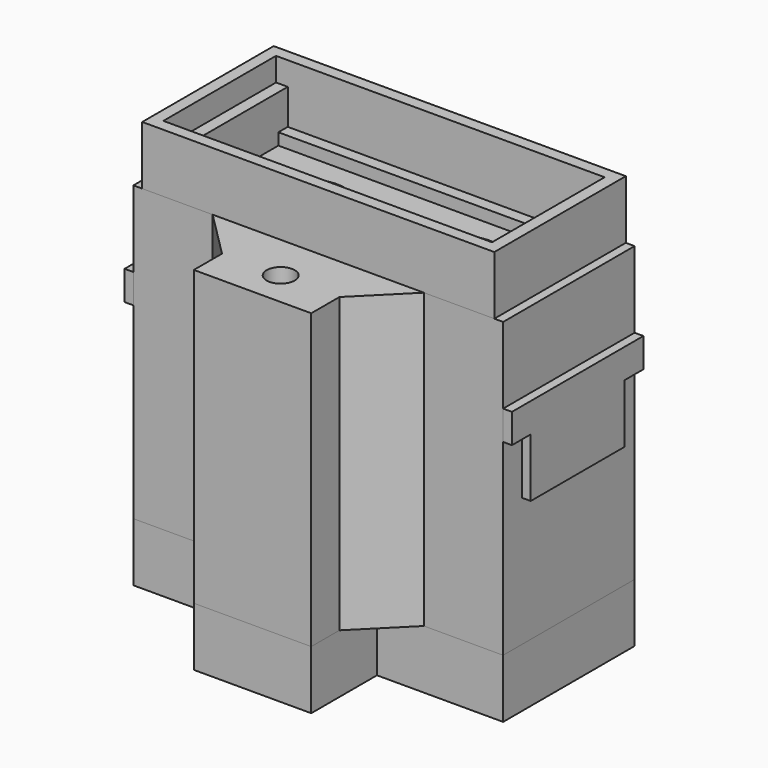
from build123d import *

# Parameters (mm, degrees)
F0_W      = 30
F0_H      = 14
F1_DEPTH  = 13
F2_W      = 30
F2_H      = 14
F2_W_2    = 28
F2_H_2    = 12
F3_DEPTH  = 6
F4_W      = 1
F4_H      = 12
F5_DEPTH  = 4
F6_R      = 3.1
F7_DEPTH  = 19
F8_W      = 1.5
F8_H      = 14
F9_DEPTH  = 7.5
F10_R     = 2.55
F11_DEPTH = 3
F13_W     = 27
F13_H     = 10
F13_W_2   = 10
F13_H_2   = 7
F14_DEPTH = 25
F15_W     = 30
F15_H     = 10
F16_DEPTH = 20
F17_R     = 1.2
F18_DEPTH = 25
F19_W     = 5
F19_H     = 5
F19_R     = 4
F19_W_2   = 10
F19_H_2   = 7
F19_R_2   = 1.5
F20_DEPTH = 5
F21_SIZE  = 4
F23_W     = 5
F23_H     = 9
F24_DEPTH = 11
F25_W     = 33
F25_H     = 2
F26_DEPTH = 5


with BuildPart() as f1:
    # F0 (on Top) → F1 (new body)
    with BuildSketch(Plane.XY):
        Rectangle(F0_W, F0_H)
    extrude(amount=F1_DEPTH)

    # F2 (on face) → F3 (join)
    with BuildSketch(Plane.XY.offset(13)):
        Rectangle(F2_W, F2_H)
        Rectangle(F2_W_2, F2_H_2, mode=Mode.SUBTRACT)
    extrude(amount=F3_DEPTH)

    # F4 (on face) → F5 (join)
    with BuildSketch(Plane.XY.offset(13)):
        with Locations((-13.5, 0)):
            Rectangle(F4_W, F4_H)
        with Locations((13.5, 0)):
            Rectangle(F4_W, F4_H)
    extrude(amount=F5_DEPTH)

    # F6 (on face) → F7 (cut)
    with BuildSketch(Plane.XY.offset(13)):
        with Locations((-6.5, 0)):
            Circle(F6_R)
        with Locations((6.5, 0)):
            Circle(F6_R)
    extrude(amount=-F7_DEPTH, mode=Mode.SUBTRACT)

    # F8 (on face) → F9 (join)
    with BuildSketch(Plane(origin=(0, 0, 0), x_dir=(1, 0, 0), z_dir=(0, 0, -1))):
        with Locations((-15.75, 0)):
            Rectangle(F8_W, F8_H)
        with Locations((15.75, 0)):
            Rectangle(F8_W, F8_H)
    extrude(amount=-F9_DEPTH)

    # F10 (on face) → F11 (cut)
    with BuildSketch(Plane(origin=(0, 0, 0), x_dir=(1, 0, 0), z_dir=(0, 0, -1))):
        Circle(F10_R)
    extrude(amount=-F11_DEPTH, mode=Mode.SUBTRACT)

    # F25 (on face) → F26 (cut)
    with BuildSketch(Plane(origin=(0, 0, 0), x_dir=(1, 0, 0), z_dir=(0, 0, -1))):
        with Locations((0, 6)):
            Rectangle(F25_W, F25_H)
        with Locations((0, -6)):
            Rectangle(F25_W, F25_H)
    extrude(amount=-F26_DEPTH, mode=Mode.SUBTRACT)


with BuildPart() as f14:
    # F13 (on offset) → F14 (new body)
    with BuildSketch(Plane.XY.offset(14)):
        Polygon((5, -7), (15.75, -7), (15.75, 7), (5, 7), (-5, 7), (-15.75, 7), (-15.75, -7), (-5, -7), align=None)
        Rectangle(F13_W, F13_H, mode=Mode.SUBTRACT)
        with Locations((0, -10.5)):
            Rectangle(F13_W_2, F13_H_2)
        with Locations((0, 10.5)):
            Rectangle(F13_W_2, F13_H_2)
    extrude(amount=-F14_DEPTH)

    # F15 (on face) → F16 (cut)
    with BuildSketch(Plane(origin=(0, 0, -11), x_dir=(1, 0, 0), z_dir=(0, 0, -1))):
        Rectangle(F15_W, F15_H)
    extrude(amount=-F16_DEPTH, mode=Mode.SUBTRACT)

    # F17 (on face) → F18 (cut)
    with BuildSketch(Plane.XY.offset(14)):
        with Locations((0, 11)):
            Circle(F17_R)
        with Locations((0, -11)):
            Circle(F17_R)
    extrude(amount=-F18_DEPTH, mode=Mode.SUBTRACT)

    # F21
    f21_edges = [f14.edges().sort_by_distance(p)[0] for p in [
        (-5, 7, 1.5),
        (5, 7, 1.5),
        (5, -7, 1.5),
        (-5, -7, 1.5),
    ]]
    chamfer(f21_edges, length=F21_SIZE)


with BuildPart() as f20:
    # F19 (on face) → F20 (new body)
    with BuildSketch(Plane(origin=(0, 0, -11), x_dir=(1, 0, 0), z_dir=(0, 0, -1))):
        Polygon((5, -7), (15.75, -7), (15.75, 7), (5, 7), (-5, 7), (-15.75, 7), (-15.75, -7), (-5, -7), align=None)
        with Locations((-7.5, 0)):
            Rectangle(F19_W, F19_H, mode=Mode.SUBTRACT)
        Circle(F19_R, mode=Mode.SUBTRACT)
        with Locations((7.5, 0)):
            Rectangle(F19_W, F19_H, mode=Mode.SUBTRACT)
        with Locations((0, -10.5)):
            Rectangle(F19_W_2, F19_H_2)
        with Locations((0, -11)):
            Circle(F19_R_2, mode=Mode.SUBTRACT)
        with Locations((0, 10.5)):
            Rectangle(F19_W_2, F19_H_2)
        with Locations((0, 11)):
            Circle(F19_R_2, mode=Mode.SUBTRACT)
    extrude(amount=F20_DEPTH)


with BuildPart() as f24:
    # F23 (on offset) → F24 (new body)
    with BuildSketch(Plane(origin=(0, 0, -11), x_dir=(1, 0, 0), z_dir=(0, 0, -1))):
        Rectangle(F23_W, F23_H)
    extrude(amount=-F24_DEPTH)


solid = Compound([f1.part, f14.part, f20.part, f24.part])
